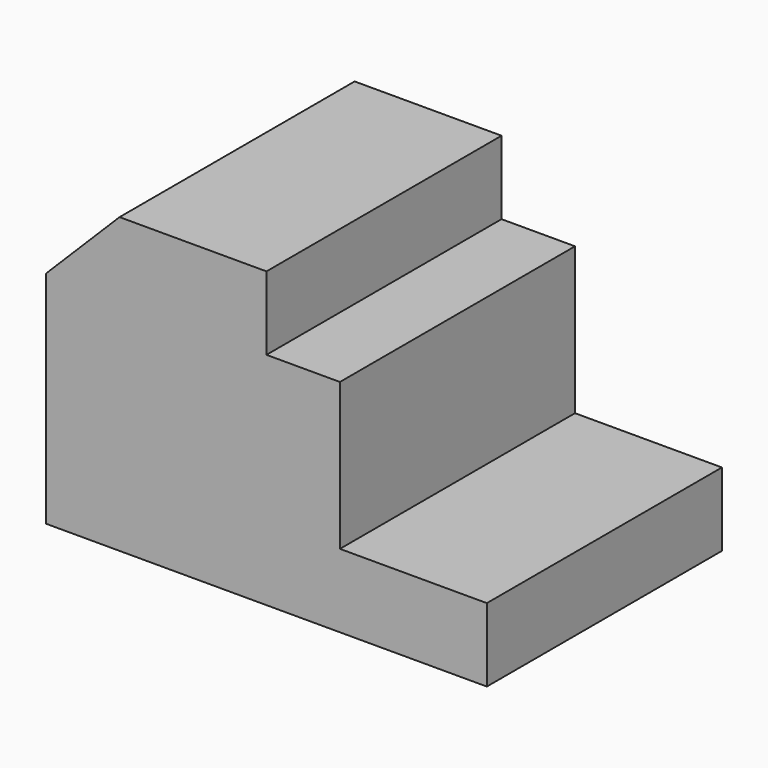
from build123d import *

# Parameters (mm, degrees)
F1_DEPTH = 25.4
F2_DEPTH = 25.4
F3_DEPTH = 12.7


# Not quite as in the source:
# - a feature names something its author has since deleted; it is built from what else it names


with BuildPart() as f1:
    # F0 (on Front) → F1 (new body, symmetric)
    with BuildSketch(Plane.XZ):
        Polygon((0, 38.1), (0, 0), (76.2, 0), (76.2, 12.7), (50.8, 12.7), (50.8, 25.4), (25.4, 25.4), (25.4, 50.8), (12.7, 50.8), align=None)
    extrude(amount=F1_DEPTH, both=True)

    # F0 (on Front) → F2 (join, symmetric)
    with BuildSketch(Plane.XZ):
        Polygon((38.1, 50.8), (25.4, 50.8), (25.4, 25.4), (50.8, 25.4), (50.8, 38.1), (38.1, 38.1), align=None)
    extrude(amount=F2_DEPTH, both=True)

    # F0 (on Front) → F3 (join, symmetric)
    with BuildSketch(Plane.XZ):
        Polygon((38.1, 50.8), (25.4, 50.8), (25.4, 25.4), (50.8, 25.4), (50.8, 38.1), (38.1, 38.1), align=None)
    extrude(amount=F3_DEPTH, both=True)


solid = f1.part
